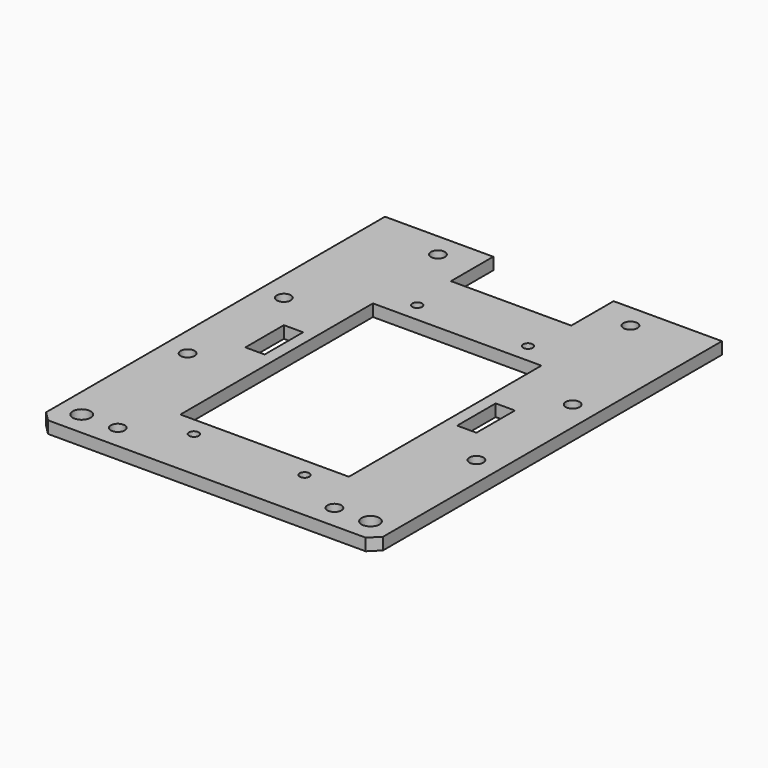
from build123d import *

# Parameters (mm, degrees)
F0_R     = 1.85
F0_R_2   = 1.45
F0_R_3   = 1
F0_W     = 35
F0_H     = 50
F0_W_2   = 4
F0_H_2   = 10
F1_DEPTH = 2.5
F2_SIZE  = 2


# Not quite as in the source:
# - a feature names something its author has since deleted; it is built from what else it names


with BuildPart() as f1:
    # F0 (on Top) → F1 (new body)
    with BuildSketch(Plane.XY):
        Polygon((-12.5, 45), (-35, 45), (-35, -45), (35, -45), (35, 45), (12.5, 45), (12.5, 34), (-12.5, 34), align=None)
        with Locations((-30, -40)):
            Circle(F0_R, mode=Mode.SUBTRACT)
        with Locations((-22.5, -40)):
            Circle(F0_R_2, mode=Mode.SUBTRACT)
        with Locations((-11.5, -34)):
            Circle(F0_R_3, mode=Mode.SUBTRACT)
        with Locations((-30, -12.5)):
            Circle(F0_R_2, mode=Mode.SUBTRACT)
        with Locations((11.5, -34)):
            Circle(F0_R_3, mode=Mode.SUBTRACT)
        with Locations((22.5, -40)):
            Circle(F0_R_2, mode=Mode.SUBTRACT)
        with Locations((30, -40)):
            Circle(F0_R, mode=Mode.SUBTRACT)
        with Locations((0, -5)):
            Rectangle(F0_W, F0_H, mode=Mode.SUBTRACT)
        with Locations((30, -12.5)):
            Circle(F0_R_2, mode=Mode.SUBTRACT)
        with Locations((-22, 0)):
            Rectangle(F0_W_2, F0_H_2, mode=Mode.SUBTRACT)
        with Locations((-30, 12.5)):
            Circle(F0_R_2, mode=Mode.SUBTRACT)
        with Locations((-20, 40)):
            Circle(F0_R_2, mode=Mode.SUBTRACT)
        with Locations((-11.5, 24)):
            Circle(F0_R_3, mode=Mode.SUBTRACT)
        with Locations((22, 0)):
            Rectangle(F0_W_2, F0_H_2, mode=Mode.SUBTRACT)
        with Locations((30, 12.5)):
            Circle(F0_R_2, mode=Mode.SUBTRACT)
        with Locations((11.5, 24)):
            Circle(F0_R_3, mode=Mode.SUBTRACT)
        with Locations((20, 40)):
            Circle(F0_R_2, mode=Mode.SUBTRACT)
    extrude(amount=-F1_DEPTH)

    # F2
    f2_edges = [f1.edges().sort_by_distance(p)[0] for p in [
        (-35, -45, -1.25),
        (35, -45, -1.25),
    ]]
    chamfer(f2_edges, length=F2_SIZE)


solid = f1.part
